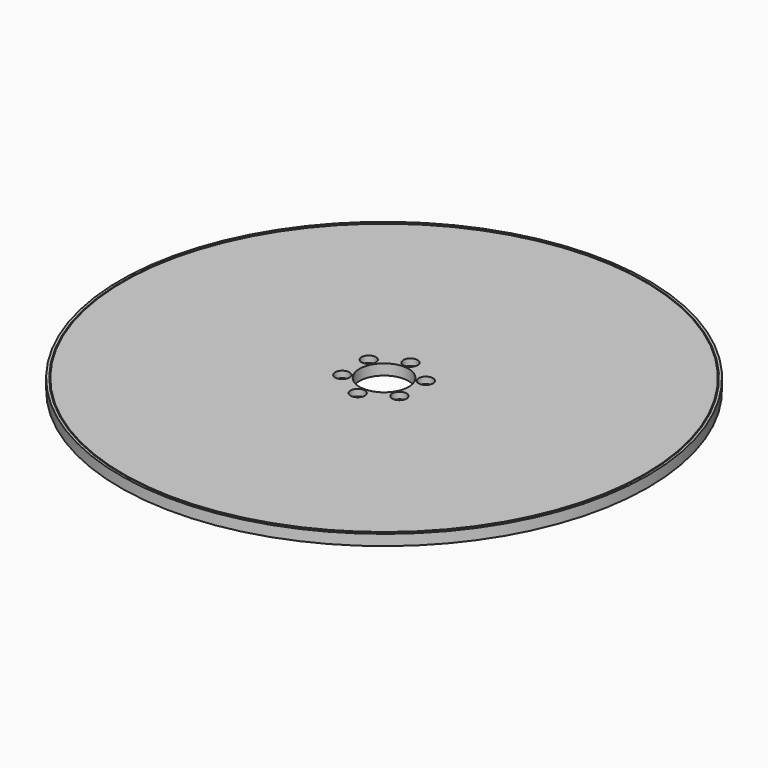
from build123d import *

# Parameters (mm, degrees)
F0_R            = 80
F1_DEPTH        = 3.3
F2_R            = 7.525
F3_DEPTH        = 3.301
F4_R            = 75
F4_R_2          = 12.5
F5_DEPTH        = 2.3
F7_D            = 2.4
F7_CBORE_D      = 4.4
F7_CBORE_DEPTH  = 2
F7_COPIES_COUNT = 6
F8_W            = 4.15
F8_H            = 10.15
F9_DEPTH        = 1.51
F10_R           = 81
F10_R_2         = 80.25
F11_DEPTH       = 3.3


# Not quite as in the source:
# - a pattern or mirror of a feature is missing from the dataset's text; its kind, count and spacing are read off the source's solid


with BuildPart() as f1:
    # F0 (on Top) → F1 (new body)
    with BuildSketch(Plane.XY):
        Circle(F0_R)
    extrude(amount=F1_DEPTH)

    # F2 (on face) → F3 (cut, through all)
    with BuildSketch(Plane(origin=(0, 0, 0), x_dir=(1, 0, 0), z_dir=(0, 0, -1))):
        Circle(F2_R)
    extrude(amount=-F3_DEPTH, mode=Mode.SUBTRACT)

    # F4 (on face) → F5 (cut)
    with BuildSketch(Plane(origin=(0, 0, 0), x_dir=(1, 0, 0), z_dir=(0, 0, -1))):
        Circle(F4_R)
        Circle(F4_R_2, mode=Mode.SUBTRACT)
    extrude(amount=-F5_DEPTH, mode=Mode.SUBTRACT)

    # F7 (through all)
    with Locations(Plane.XY.offset(3.3)):
        with Locations((0, -10.125)):
            f7 = CounterBoreHole(F7_D / 2, F7_CBORE_D / 2, F7_CBORE_DEPTH)

    # F7_copies: F7 ×6 about axis
    f7_copies_axis = Axis((0, 0, 0), (0, 0, 1))
    for i in range(1, F7_COPIES_COUNT):
        add(f7.rotate(f7_copies_axis, i * 360 / F7_COPIES_COUNT), mode=Mode.SUBTRACT)

    # F8 (on face) → F9 (cut)
    with BuildSketch(Plane(origin=(0, 0, 0), x_dir=(1, 0, 0), z_dir=(0, 0, -1))):
        with Locations((-76.9030988333, 0)):
            Rectangle(F8_W, F8_H)
    f9 = extrude(amount=-F9_DEPTH, mode=Mode.SUBTRACT)

    # F9_copies: F9 across plane
    add(f9.mirror(Plane(origin=(0, 0, 0), x_dir=(0, 0, 1), z_dir=(1, 0, 0))), mode=Mode.SUBTRACT)


with BuildPart() as f11:
    # F10 (on face) → F11 (new body)
    with BuildSketch(Plane.XY.offset(3.3)):
        Circle(F10_R)
        Circle(F10_R_2, mode=Mode.SUBTRACT)
    extrude(amount=-F11_DEPTH)


solid = Compound([f1.part, f11.part])
